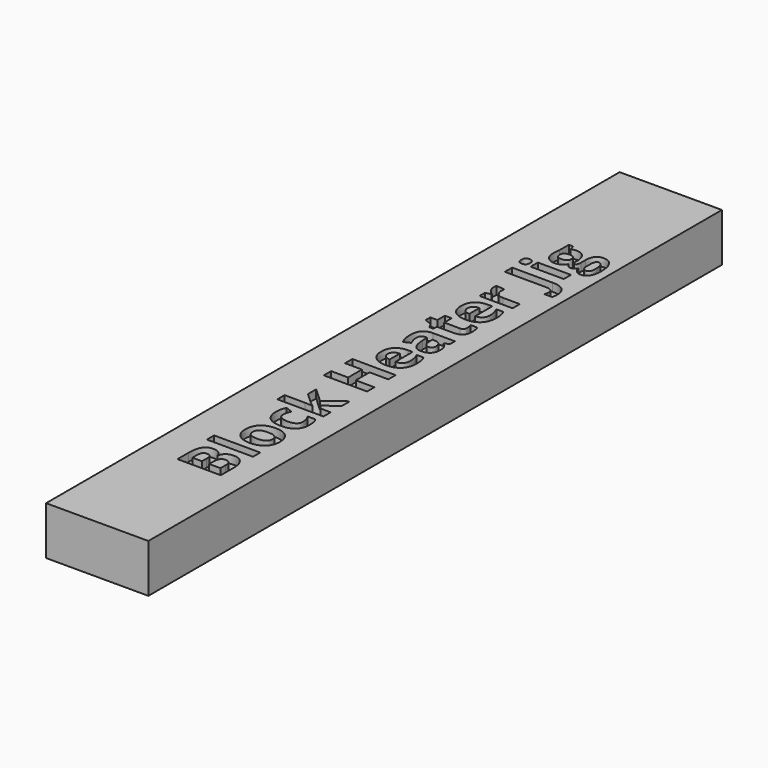
from build123d import *

# Parameters (mm, degrees)
F0_W         = 12.7
F0_H         = 89
F1_DEPTH     = 6
F2_TEXT_SIZE = 7.5532563583
F3_DEPTH     = 1


# Not quite as in the source:
# - Text() gives the source's letters only with a copy of the font that has no kerning and outlines rounded to 1/6400 em; it was checked with that copy


with BuildPart() as f1:
    # F0 (on Top) → F1 (new body)
    with BuildSketch(Plane.XY):
        with Locations((6.35, 44.5)):
            Rectangle(F0_W, F0_H)
    extrude(amount=F1_DEPTH)

    # F2 (on face) → F3 (cut)
    with BuildSketch(Plane.XY.offset(6)):
        with Locations(Location((9.549403093, 14.4764996215), (0, 0, 89.7493870421))):
            Text('Block Heater Jig', F2_TEXT_SIZE, font='Open Sans', font_style=FontStyle.BOLD, text_align=(TextAlign.LEFT, TextAlign.BOTTOM))
    extrude(amount=-F3_DEPTH, mode=Mode.SUBTRACT)


solid = f1.part
